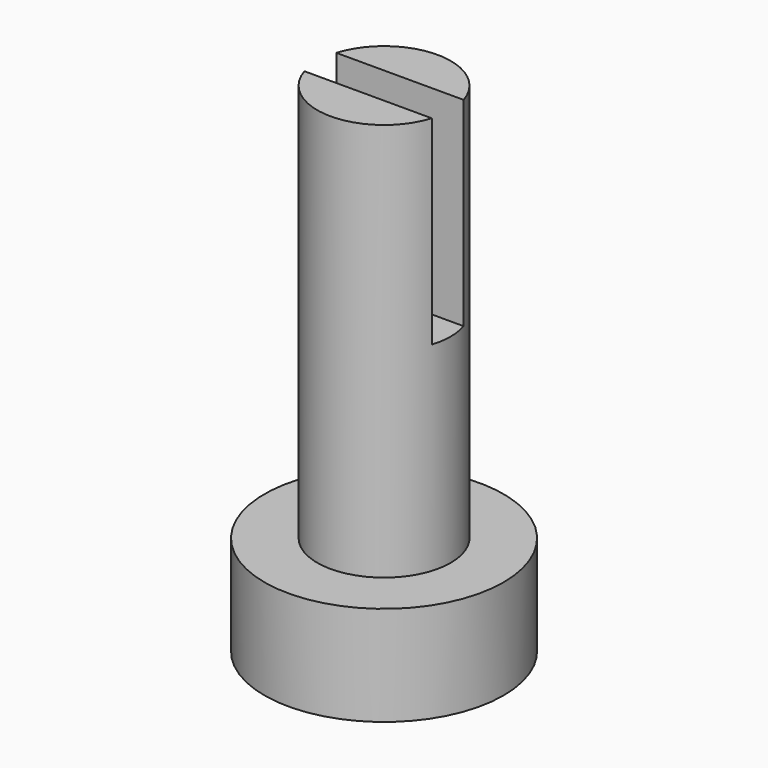
from build123d import *

# Parameters (mm, degrees)
F0_R     = 3.35
F1_DEPTH = 25
F0_R_2   = 6
F2_DEPTH = 5
F4_DEPTH = 10


with BuildPart() as f1:
    # F0 (on Top) → F1 (new body)
    with BuildSketch(Plane.XY):
        Circle(F0_R)
    extrude(amount=F1_DEPTH)

    # F0 (on Top) → F2 (join)
    with BuildSketch(Plane.XY):
        Circle(F0_R_2)
        Circle(F0_R, mode=Mode.SUBTRACT)
    extrude(amount=F2_DEPTH)

    # F3 (on face) → F4 (cut)
    with BuildSketch(Plane.XY.offset(25)):
        with BuildLine():
            ThreePointArc((-3.1972644557, 1), (-3.35, 0), (-3.1972644557, -1))
            Line((-3.1972644557, -1), (3.1972644557, -1))
            ThreePointArc((3.1972644557, -1), (3.3115959843, -0.505798415), (3.35, 0))
            ThreePointArc((3.35, 0), (3.3115959843, 0.505798415), (3.1972644557, 1))
            Line((3.1972644557, 1), (-3.1972644557, 1))
        make_face()
    extrude(amount=-F4_DEPTH, mode=Mode.SUBTRACT)


solid = f1.part
